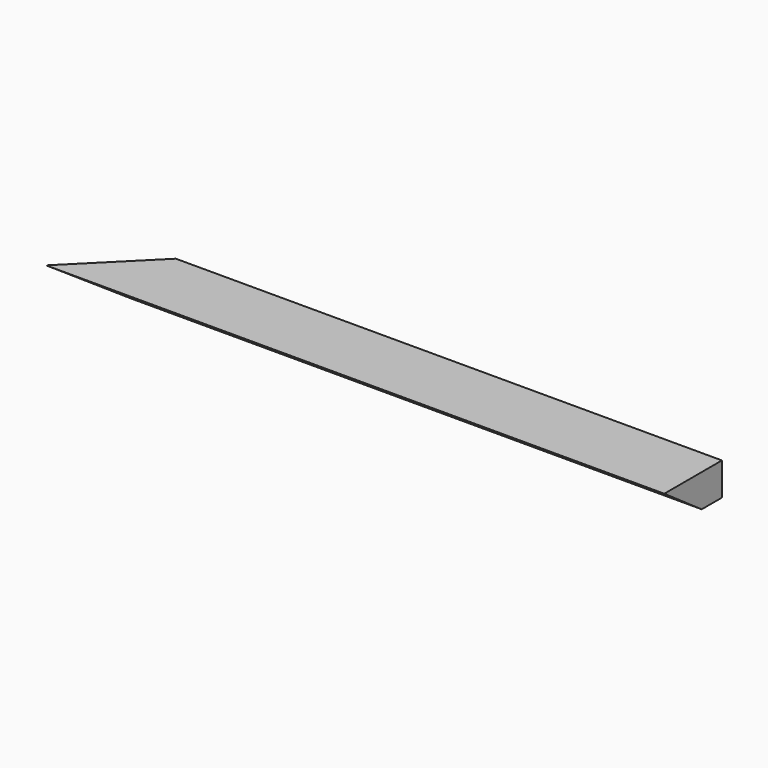
from build123d import *

# Parameters (mm, degrees)
F1_DEPTH      = 228.6
F1_DEPTH_BACK = 228.6
F3_DEPTH      = 19.051


# Not quite as in the source:
# - a feature names something its author has since deleted; it is built from what else it names


with BuildPart() as f1:
    # F0 (on Right) → F1 (new body, two sides)
    with BuildSketch(Plane.YZ) as f1_sk:
        Polygon((0, 0), (0, 19.05), (-41.91, 19.05), (-14.7037804716, 0), align=None)
    extrude(amount=F1_DEPTH)
    extrude(f1_sk.sketch, amount=-F1_DEPTH_BACK)

    # F2 (on Top) → F3 (cut, through all)
    with BuildSketch(Plane.XY):
        Polygon((-237.7350770505, -148.8350770505), (-88.9, 0), (-237.7350770505, 0), align=None)
    extrude(amount=F3_DEPTH, mode=Mode.SUBTRACT)


solid = f1.part
